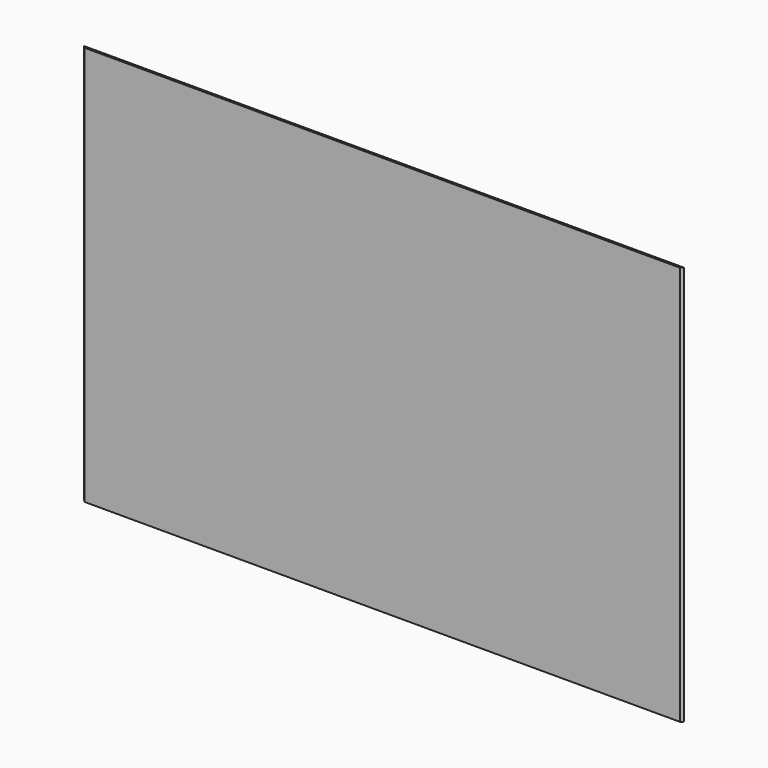
from build123d import *

# Parameters (mm, degrees)
F0_W     = 1828.8
F0_H     = 1219.2
F1_DEPTH = 3.175
F2_SIZE  = 6.34999
F3_SIZE  = 6.34999


# Not quite as in the source:
# - a fillet or chamfer is up to 0.001 mm smaller than in the source, because OpenCascade refuses the exact size


with BuildPart() as f1:
    # F0 (on Front) → F1 (new body, symmetric)
    with BuildSketch(Plane.XZ):
        Rectangle(F0_W, F0_H)
    extrude(amount=F1_DEPTH, both=True)

    # F2 (size 6.35 in the source; OpenCascade refuses exactly that, so slightly less here)
    f2_edges = [f1.edges().sort_by_distance(p)[0] for p in [
        (-914.4, -3.175, 0),
    ]]
    chamfer(f2_edges, length=F2_SIZE)

    # F3 (size 6.35 in the source; OpenCascade refuses exactly that, so slightly less here)
    f3_edges = [f1.edges().sort_by_distance(p)[0] for p in [
        (914.4, -3.175, 0),
    ]]
    chamfer(f3_edges, length=F3_SIZE)


solid = f1.part
